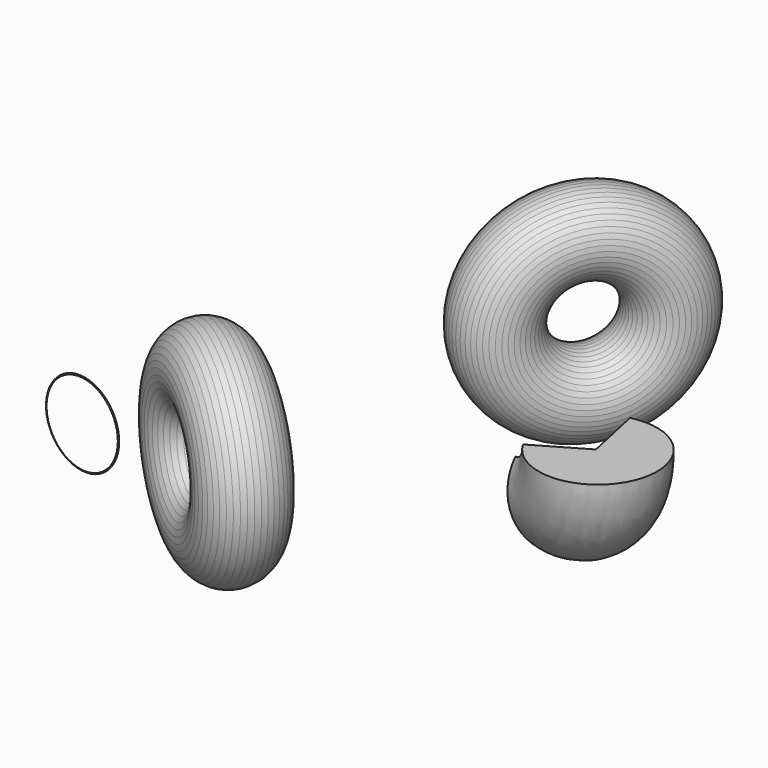
from build123d import *

# Parameters (mm, degrees)
F5_ANGLE = 80


with BuildPart() as f1:
    # F0 (on Top) → F1 (revolve)
    with BuildSketch(Plane.XY):
        Polygon((-1.9237758445, 28.0432676629), (1.9237758445, 32.8317458078), (5.0674560726, 38.1090985122), (7.4460766801, 43.7726081086), (9.0133405225, 49.7120408249), (9.7387425919, 55.8117923592), (9.6081637621, 61.9531379864), (8.6241456014, 68.0165433994), (6.8058409042, 73.883991309), (4.188640903, 79.4412785156), (0.8234864188, 84.5802387451), (-3.2241236441, 89.2008479822), (-7.87540716, 93.2131713239), (-13.039832186, 96.5391134602), (-18.6168790633, 99.1139387108), (-24.4979969184, 100.887531031), (-30.5687164818, 101.8253694636), (-36.7108781026, 101.9092000503), (-42.8049315914, 101.1373911242), (-48.732263129, 99.524965068), (-54.3775039492, 97.1033059208), (-59.6307758609, 93.9195485234), (-64.3898299017, 90.035661092), (-68.5620364981, 85.5272390776), (-72.0661883946, 80.4820337864), (-74.8340812603, 74.9982444007), (-76.8118412091, 69.1826066431), (-77.9609733932, 63.1483152873), (-78.2591112619, 57.0128209507), (-77.7004519005, 50.8955440515), (-76.2958689782, 44.9155504263), (-74.0727011037, 39.1892338488), (-71.074219711, 33.8280505577), (-67.3587868297, 28.9363498874), (-62.9987191346, 24.6093432273), (-58.0788803837, 20.9312508401), (-52.6950296422, 17.9736626103), (-46.9519574408, 15.7941446287), (-40.9614461471, 14.4351187336), (-34.8400942495, 13.9230368181), (-28.7070468995, 14.2678659743), (-22.6816768878, 15.4628944949), (-16.8812611878, 17.484862509), (-11.4186982932, 20.2944147092), (-6.4003107772, 23.8368663578), align=None)
    revolve(axis=Axis((39.8637475446, 35.3185385466, 0), (-0.559472867, -0.828848666, 0)))


with BuildPart() as f3:
    # F2 (on Top) → F3 (revolve)
    with BuildSketch(Plane.XY):
        with BuildLine():
            add(Edge.make_bspline(
                [(-51.4495074749, -19.7882745415), (-50.9200883915, -19.8398778668), (-50.493013893, -19.7362751838), (-50.1684964465, -19.505778796)],
                knots=[0.7757199217, 0.7757199217, 0.7757199217, 0.7757199217, 0.8167471148, 0.8167471148, 0.8167471148, 0.8167471148], degree=3))
            ThreePointArc((-50.1684964465, -19.505778796), (-50.8098662967, -19.643107233), (-51.4495074749, -19.7882745415))
        make_face()
    revolve(axis=Axis((-99.6861457825, -43.7775719911, 0), (0.1416418581, 0.9899179683, 0)))


with BuildPart() as f5:
    # F4 (on Top) → F5 (revolve)
    with BuildSketch(Plane.XY):
        with BuildLine():
            Line((276.3892473231, 223.0473164586), (221.9546566931, 191.4982249494))
            ThreePointArc((221.9546566931, 191.4982249494), (337.3997552126, 198.5504997973), (262.5981761207, 286.7663097072))
            Line((262.5981761207, 286.7663097072), (276.3892473231, 223.0473164586))
        make_face()
    revolve(axis=Axis((225.1779809594, 239.2845153809, 0), (0.4675932683, 0.88394374, 0)), revolution_arc=F5_ANGLE)


with BuildPart() as f7:
    # F6 (on Top) → F7 (revolve)
    with BuildSketch(Plane.XY):
        Polygon((86.7284355387, 388.7271249301), (81.9460526109, 391.419172287), (76.8639772007, 393.4906005299), (71.5623566734, 394.9087419981), (66.1248007515, 395.6512317534), (60.6370629403, 395.7063602888), (55.1856881432, 395.0732581945), (49.8566477974, 393.7619098685), (44.7339840523, 391.7929960575), (39.8984843756, 389.1975677083), (35.4264074855, 386.0165562764), (31.3882807062, 382.3001282125), (27.8477877093, 378.1068938071), (24.8607641843, 373.5029828717), (22.4743172765, 368.561001832), (20.7260826793, 363.3588886813), (19.6436310967, 357.9786838514), (19.2440334366, 352.5052363866), (19.5335915929, 347.0248658231), (20.5077390606, 341.6240008783), (22.1511129521, 336.3878164189), (24.4377962794, 331.3988902018), (27.3317266805, 326.7359005735), (30.7872651442, 322.472385666), (34.7499157647, 318.6755836565), (39.1571851746, 315.4053723806), (43.9395681024, 312.7133250237), (49.0216435125, 310.6418967807), (54.3232640399, 309.2237553125), (59.7608199617, 308.4812655572), (65.2485577729, 308.4261370218), (70.69993257, 309.0592391162), (76.0289729159, 310.3705874421), (81.1516366609, 312.3395012532), (85.9871363377, 314.9349296024), (90.4592132277, 318.1159410342), (94.497340007, 321.8323690981), (98.0378330039, 326.0256035036), (101.0248565289, 330.6295144389), (103.4113034367, 335.5714954786), (105.1595380339, 340.7736086293), (106.2419896166, 346.1538134592), (106.6415872766, 351.627260924), (106.3520291203, 357.1076314876), (105.3778816526, 362.5084964323), (103.7345077612, 367.7446808917), (101.4478244338, 372.7336071089), (98.5538940327, 377.3965967372), (95.098355569, 381.6601116446), (91.1357049485, 385.4569136542), align=None)
    revolve(axis=Axis((113.7847863138, 411.5575104952, 0), (0.8131039454, -0.5821185223, 0)))


solid = Compound([f1.part, f3.part, f5.part, f7.part])
